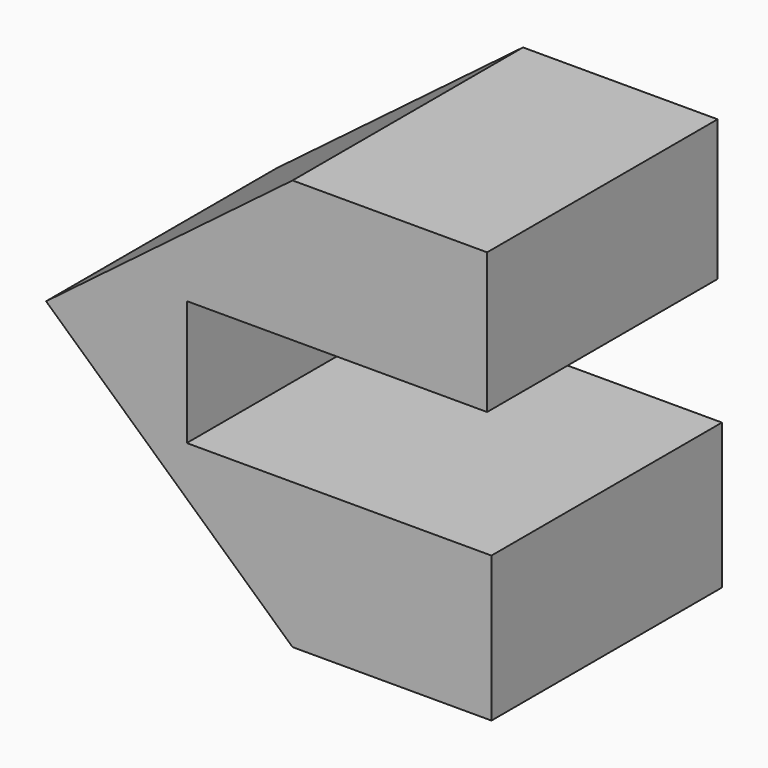
from build123d import *

# Parameters (mm, degrees)
F1_DEPTH      = 25
F1_DEPTH_BACK = 25


with BuildPart() as f1:
    # F0 (on Front) → F1 (new body, two sides)
    with BuildSketch(Plane.XZ) as f1_sk:
        Polygon((-42.7725724876, 38.9332138002), (0, 0), (34.5220863819, 0), (34.5220863819, 25.2119097859), (-18.3541122824, 25.2119097859), (-18.3541122824, 46.9000972807), (33.7701886892, 46.9000972807), (33.7701886892, 71.300983429), (0, 71.300983429), align=None)
    extrude(amount=-F1_DEPTH)
    extrude(f1_sk.sketch, amount=F1_DEPTH_BACK)


solid = f1.part
